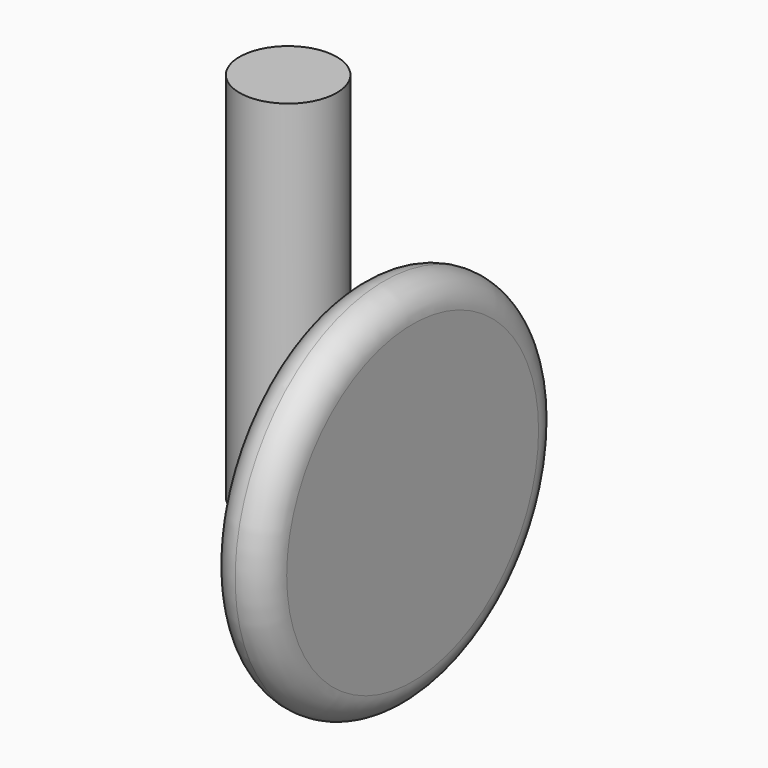
from build123d import *

# Parameters (mm, degrees)
F0_R     = 43.18
F1_DEPTH = 330.2
F3_DEPTH = 71.12
F4_R     = 19.05
F5_DEPTH = 76.2
F6_R     = 165.1
F6_R_2   = 19.05
F7_DEPTH = 50.8
F8_R     = 25.39999


# Not quite as in the source:
# - a fillet or chamfer is up to 0.001 mm smaller than in the source, because OpenCascade refuses the exact size


with BuildPart() as f1:
    # F0 (on Top) → F1 (new body)
    with BuildSketch(Plane.XY):
        Circle(F0_R)
    extrude(amount=F1_DEPTH)

    # F2 (on face) → F3 (cut)
    with BuildSketch(Plane(origin=(0, 0, 0), x_dir=(1, 0, 0), z_dir=(0, 0, -1))):
        with BuildLine():
            ThreePointArc((43.18, 0), (40.8909417637, 13.8723927885), (34.2664621733, 26.2739789549))
            Line((34.2664621733, 26.2739789549), (34.2664621733, -26.2739789549))
            ThreePointArc((34.2664621733, -26.2739789549), (40.8909417637, -13.8723927885), (43.18, 0))
        make_face()
    extrude(amount=-F3_DEPTH, mode=Mode.SUBTRACT)

    # F4 (on face) → F5 (join)
    with BuildSketch(Plane.YZ.offset(34.2664621733)):
        with Locations((0, 31.7187957861)):
            Circle(F4_R)
    extrude(amount=F5_DEPTH)

    # F6 (on face) → F7 (join)
    with BuildSketch(Plane.YZ.offset(110.4664621733)):
        with Locations((0, 31.7187957861)):
            Circle(F6_R)
        with Locations((0, 31.7187957861)):
            Circle(F6_R_2, mode=Mode.SUBTRACT)
    extrude(amount=-F7_DEPTH)

    # F8 (radius 25.4 in the source; OpenCascade refuses exactly that, so slightly less here)
    f8_edges = [f1.edges().sort_by_distance(p)[0] for p in [
        (110.466462, -165.1, 31.718796),
        (59.666462, -165.1, 31.718796),
    ]]
    fillet(f8_edges, radius=F8_R)


solid = f1.part
